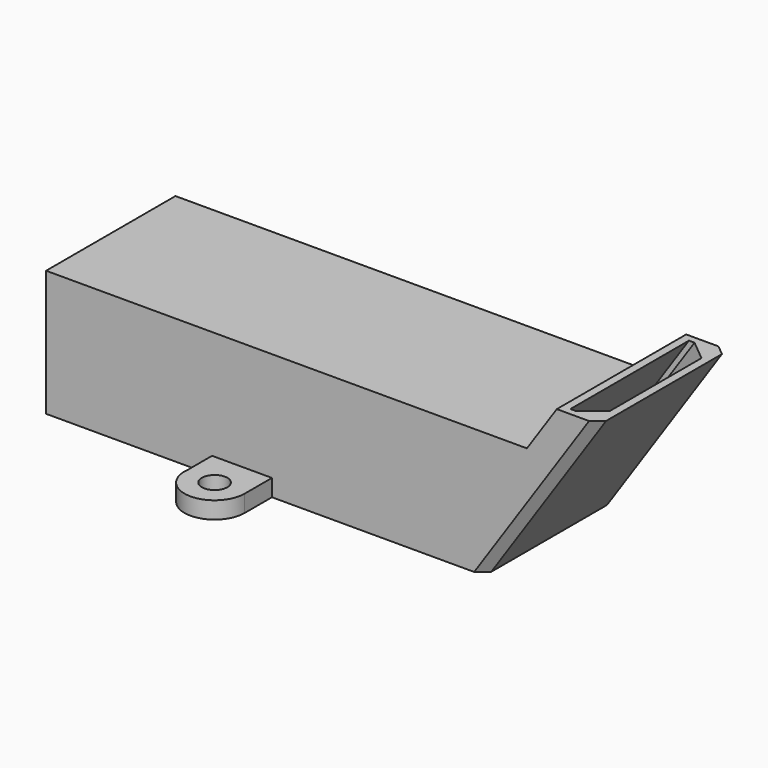
from build123d import *

# Parameters (mm, degrees)
F2_DEPTH = 9.5
F3_T     = -0.8
F4_R     = 5
F5_SIZE  = 2
F0_R     = 1.5
F6_DEPTH = 2
F7_SIZE  = 1


with BuildPart() as f2:
    # F1 (on Front) → F2 (new body, symmetric)
    with BuildSketch(Plane.XZ):
        Polygon((-24, 0), (27.5, 0), (41, 20), (36, 20), (32.49, 14.8), (-24, 14.8), align=None)
    extrude(amount=F2_DEPTH, both=True)

    # F3
    f3_openings = [f2.faces().sort_by_distance(p)[0] for p in [
        (-24, 0, 7.4),
        (38.5, 0, 20),
    ]]
    offset(amount=F3_T, openings=f3_openings, kind=Kind.INTERSECTION)

    # F4
    f4_edges = [f2.edges().sort_by_distance(p)[0] for p in [
        (27.074806, 0, 0.8),
    ]]
    fillet(f4_edges, radius=F4_R)

    # F5
    f5_edges = [f2.edges().sort_by_distance(p)[0] for p in [
        (4.457597, -8.7, 14),
        (4.457597, 8.7, 14),
        (0.208671, 8.7, 0.8),
        (0.208671, -8.7, 0.8),
        (26.763954, 8.7, 1.384866),
        (34.298195, 8.7, 11.501318),
        (26.763954, -8.7, 1.384866),
        (34.298195, -8.7, 11.501318),
    ]]
    chamfer(f5_edges, length=F5_SIZE)

    # F0 (on Top) → F6 (join)
    with BuildSketch(Plane.XY):
        with BuildLine():
            Line((2.5, -9.5), (-4.5, -9.5))
            Line((-4.5, -9.5), (-4.5, -13))
            ThreePointArc((-4.5, -13), (-1.2506305341, -17.0266392409), (2.5355339059, -13.5))
            Line((2.5355339059, -13.5), (2.5355339059, -9.5))
            Line((2.5355339059, -9.5), (2.5, -9.5))
        make_face()
        with Locations((-1, -13.5)):
            Circle(F0_R, mode=Mode.SUBTRACT)
        with BuildLine():
            Line((-4.5, 13), (-4.5, 9.5))
            Line((-4.5, 9.5), (2.5, 9.5))
            Line((2.5, 9.5), (2.5355339059, 9.5))
            Line((2.5355339059, 9.5), (2.5355339059, 13.5))
            ThreePointArc((2.5355339059, 13.5), (-1.2506305341, 17.0266392409), (-4.5, 13))
        make_face()
        with Locations((-1, 13.5)):
            Circle(F0_R, mode=Mode.SUBTRACT)
    extrude(amount=F6_DEPTH)

    # F7
    f7_edges = [f2.edges().sort_by_distance(p)[0] for p in [
        (34.25, 9.5, 10),
        (34.25, -9.5, 10),
    ]]
    chamfer(f7_edges, length=F7_SIZE)


solid = f2.part
